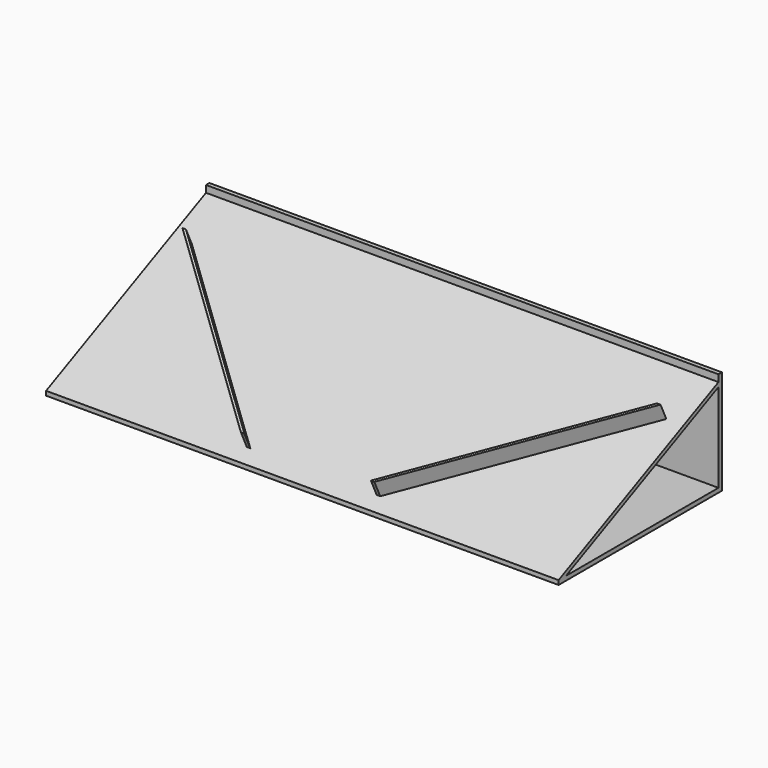
from build123d import *

# Parameters (mm, degrees)
F1_W     = 2974
F1_H     = 1185
F2_DEPTH = 25
F3_W     = 2974
F3_H     = 25
F4_DEPTH = 580
F6_DEPTH = 2974
F8_DEPTH = 100


with BuildPart() as f2:
    # F1 (on Top) → F2 (new body)
    with BuildSketch(Plane.XY):
        with Locations((1487, 592.5)):
            Rectangle(F1_W, F1_H)
    extrude(amount=F2_DEPTH)

    # F3 (on face) → F4 (join)
    with BuildSketch(Plane.XY.offset(25)):
        with Locations((1487, 1172.5)):
            Rectangle(F3_W, F3_H)
    extrude(amount=F4_DEPTH)

    # F5 (on Right) → F6 (join)
    with BuildSketch(Plane.YZ):
        Polygon((1160, 540), (1160, 565), (0, 25), (53.7037037037, 25), align=None)
    extrude(amount=F6_DEPTH)

    # F7 (on face) → F8 (join)
    with BuildSketch(Plane(origin=(0, -9.5651111654, 20.5472758368), x_dir=(1, 0, 0), z_dir=(0, -0.4220295802, 0.9065820611))):
        Polygon((120, 1010.5507395039), (100, 1010.5507395039), (1100, 100), (1120, 100), align=None)
        Polygon((1874, 100), (2874, 1010.5507395039), (2854, 1010.5507395039), (1854, 100), align=None)
    extrude(amount=F8_DEPTH)


solid = f2.part
